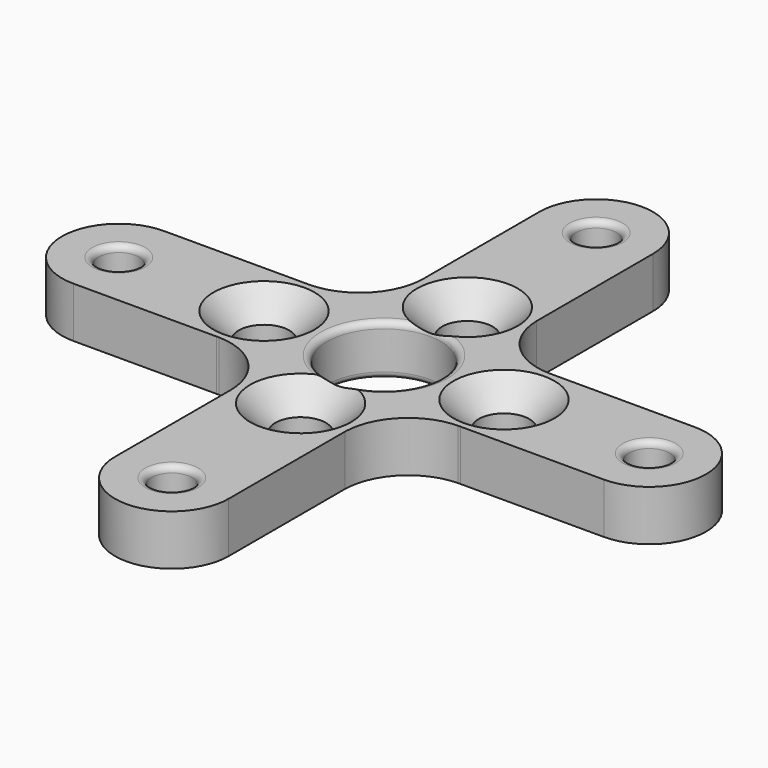
from build123d import *

# Parameters (mm, degrees)
F1_DEPTH = 4
F2_R     = 4.5
F3_DEPTH = 4.001
F4_R     = 1.6
F5_DEPTH = 4.001
F6_R     = 2
F7_DEPTH = 4.001
F8_R     = 0.5


# Not quite as in the source:
# - a fillet or chamfer that OpenCascade refuses, or shapes differently, is made with other operations: its cross-section is extruded or revolved along the edge and cut away or added


with BuildPart() as f1:
    # F0 (on Top) → F1 (new body)
    with BuildSketch(Plane.XY):
        with BuildLine():
            Line((4.5, -21), (4.5, -9.4618145376))
            ThreePointArc((4.5, -9.4618145376), (5.9839541329, -5.9839541329), (9.4618145376, -4.5))
            ThreePointArc((9.4618145376, -4.5), (9.5692863688, -4.4988608952), (9.6767581999, -4.5))
            Line((9.6767581999, -4.5), (21, -4.5))
            ThreePointArc((21, -4.5), (25.5, 0), (21, 4.5))
            Line((21, 4.5), (9.6767581999, 4.5))
            ThreePointArc((9.6767581999, 4.5), (9.5692863688, 4.4988608952), (9.4618145376, 4.5))
            ThreePointArc((9.4618145376, 4.5), (5.9839541329, 5.9839541329), (4.5, 9.4618145376))
            Line((4.5, 9.4618145376), (4.5, 21))
            ThreePointArc((4.5, 21), (0, 25.5), (-4.5, 21))
            Line((-4.5, 21), (-4.5, 9.4618145376))
            ThreePointArc((-4.5, 9.4618145376), (-5.9839541329, 5.9839541329), (-9.4618145376, 4.5))
            ThreePointArc((-9.4618145376, 4.5), (-9.5692863688, 4.4988608952), (-9.6767581999, 4.5))
            Line((-9.6767581999, 4.5), (-21, 4.5))
            ThreePointArc((-21, 4.5), (-25.5, 0), (-21, -4.5))
            Line((-21, -4.5), (-9.6767581999, -4.5))
            ThreePointArc((-9.6767581999, -4.5), (-9.5692863688, -4.4988608952), (-9.4618145376, -4.5))
            ThreePointArc((-9.4618145376, -4.5), (-5.9839541329, -5.9839541329), (-4.5, -9.4618145376))
            Line((-4.5, -9.4618145376), (-4.5, -21))
            ThreePointArc((-4.5, -21), (0, -25.5), (4.5, -21))
        make_face()
    extrude(amount=F1_DEPTH)

    # F2 (on face) → F3 (cut, through all)
    with BuildSketch(Plane.XY.offset(4)):
        Circle(F2_R)
    extrude(amount=-F3_DEPTH, mode=Mode.SUBTRACT)

    # F4 (on face) → F5 (cut, through all)
    with BuildSketch(Plane.XY.offset(4)):
        with Locations((21, 0)):
            Circle(F4_R)
        with Locations((0, -21)):
            Circle(F4_R)
        with Locations((-21, 0)):
            Circle(F4_R)
        with Locations((0, 21)):
            Circle(F4_R)
    extrude(amount=-F5_DEPTH, mode=Mode.SUBTRACT)

    # F6 (on Top) → F7 (cut, through all)
    with BuildSketch(Plane.XY):
        with Locations((9.5, 0)):
            Circle(F6_R)
        with Locations((-9.5, 0)):
            Circle(F6_R)
        with Locations((0, -8.25)):
            Circle(F6_R)
        with Locations((0, 8.25)):
            Circle(F6_R)
    extrude(amount=F7_DEPTH, mode=Mode.SUBTRACT)

    # F8
    f8_edges = [f1.edges().sort_by_distance(p)[0] for p in [
        (-4.5, 0, 4),
        (-4.5, 0, 0),
        (19.4, 0, 4),
        (-22.6, 0, 4),
        (-1.6, -21, 4),
        (-1.6, 21, 4),
        (-22.6, 0, 0),
        (19.4, 0, 0),
        (-1.6, 21, 0),
        (-1.6, -21, 0),
    ]]
    fillet(f8_edges, radius=F8_R)

    # F9: chamfer of 2 on 4 edges, made by hand

    # F9_s1 → F9_t2 (revolve, cut)
    with BuildSketch(Plane.XZ.offset(-8.25)):
        Polygon((2, 2), (4, 4), (2, 4), align=None)
    revolve(axis=Axis((0, 8.25, 4), (0, 0, -1)), mode=Mode.SUBTRACT)

    # F9_s3 → F9_t4 (revolve, cut)
    with BuildSketch(Plane.XZ):
        Polygon((11.5, 2), (13.5, 4), (11.5, 4), align=None)
    revolve(axis=Axis((9.5, 0, 4), (0, 0, -1)), mode=Mode.SUBTRACT)

    # F9_s5 → F9_t6 (revolve, cut)
    with BuildSketch(Plane.XZ.offset(8.25)):
        Polygon((2, 2), (4, 4), (2, 4), align=None)
    revolve(axis=Axis((0, -8.25, 4), (0, 0, -1)), mode=Mode.SUBTRACT)

    # F9_s7 → F9_t8 (revolve, cut)
    with BuildSketch(Plane.XZ):
        Polygon((-7.5, 2), (-5.5, 4), (-7.5, 4), align=None)
    revolve(axis=Axis((-9.5, 0, 4), (0, 0, -1)), mode=Mode.SUBTRACT)


solid = f1.part
